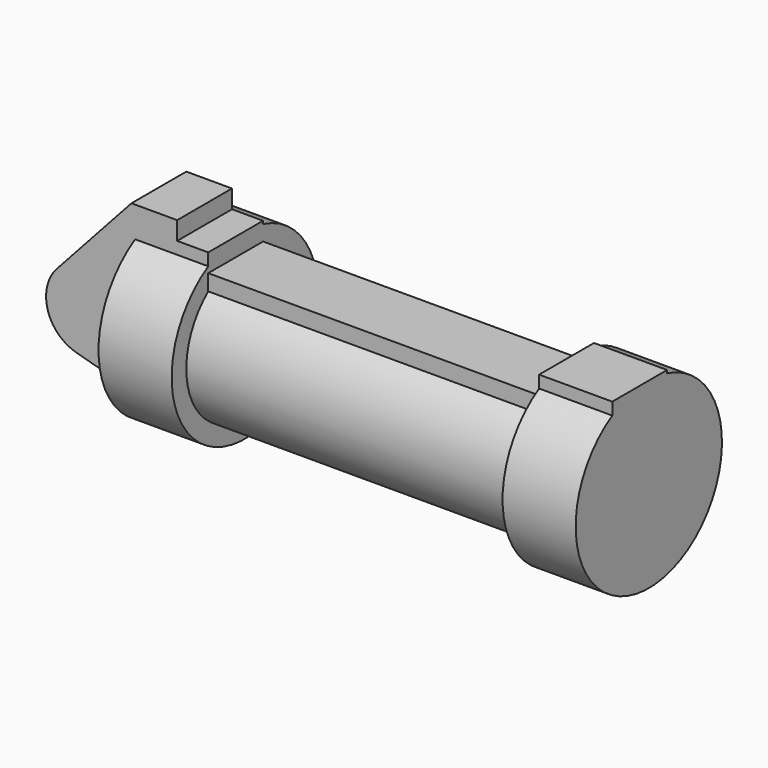
from build123d import *

# Parameters (mm, degrees)
F0_W     = 5.842
F0_H     = 12.7
F0_R     = 3.175
F2_DEPTH = 6.35
F3_DEPTH = 6.35
F4_DEPTH = 3.175
F5_DEPTH = 3.175


# Not quite as in the source:
# - the program builds the solid bodies; features that only make, move or delete a surface that nothing else refers to are left out


with BuildPart() as f1:
    # F0 (on Front) → F1 (revolve)
    with BuildSketch(Plane.XZ):
        Polygon((5.842, 12.7), (5.842, 0), (66.294, 0), (66.294, 12.7), (56.134, 12.7), (56.134, 10.16), (10.16, 10.16), (10.16, 12.7), align=None)
        with Locations((2.921, 6.35)):
            Rectangle(F0_W, F0_H)
    revolve(axis=Axis((33.147, 0, 0), (-1, 0, 0)))

    # F0 (on Front) → F2 (join)
    with BuildSketch(Plane.XZ):
        Polygon((5.842, 12.7), (5.842, 0), (66.294, 0), (66.294, 12.7), (56.134, 12.7), (56.134, 10.16), (10.16, 10.16), (10.16, 12.7), align=None)
        with BuildLine():
            ThreePointArc((-8.1826630726, -5.5069827884), (-3.1957909266, -4.5493385486), (-0.9398, 0))
            ThreePointArc((-0.9398, 0), (-4.5919612295, 5.3297205562), (-10.8806298187, 3.8475430269))
            ThreePointArc((-10.8806298187, 3.8475430269), (-12.1459778134, -1.5837270034), (-8.1826630726, -5.5069827884))
        make_face()
        with Locations((-6.6548, 0)):
            Circle(F0_R, mode=Mode.SUBTRACT)
        with Locations((2.921, 6.35)):
            Rectangle(F0_W, F0_H)
        with BuildLine():
            Line((5.842, 0), (0, 0))
            Line((0, 0), (-0.9398, 0))
            ThreePointArc((-0.9398, 0), (-3.1957909266, -4.5493385486), (-8.1826630726, -5.5069827884))
            Line((-8.1826630726, -5.5069827884), (5.842, -9.398))
            Line((5.842, -9.398), (5.842, 0))
        make_face()
        with Locations((-6.6548, 0)):
            Circle(F0_R)
    extrude(amount=F2_DEPTH)

    # F0 (on Front) → F3 (join)
    with BuildSketch(Plane.XZ):
        with BuildLine():
            Line((-0.9398, 0), (0, 0))
            Line((0, 0), (0, 12.7))
            Line((0, 12.7), (5.842, 12.7))
            Line((5.842, 12.7), (5.842, 15.24))
            Line((5.842, 15.24), (-0.508, 15.24))
            Line((-0.508, 15.24), (-10.8806298187, 3.8475430269))
            ThreePointArc((-10.8806298187, 3.8475430269), (-4.5919612295, 5.3297205562), (-0.9398, 0))
        make_face()
    extrude(amount=F3_DEPTH)

    # F0 (on Front) → F4 (join, symmetric)
    with BuildSketch(Plane.XZ):
        with BuildLine():
            Line((-0.9398, 0), (0, 0))
            Line((0, 0), (0, 12.7))
            Line((0, 12.7), (5.842, 12.7))
            Line((5.842, 12.7), (5.842, 15.24))
            Line((5.842, 15.24), (-0.508, 15.24))
            Line((-0.508, 15.24), (-10.8806298187, 3.8475430269))
            ThreePointArc((-10.8806298187, 3.8475430269), (-4.5919612295, 5.3297205562), (-0.9398, 0))
        make_face()
        with Locations((2.921, 6.35)):
            Rectangle(F0_W, F0_H)
        with BuildLine():
            Line((5.842, 0), (0, 0))
            Line((0, 0), (-0.9398, 0))
            ThreePointArc((-0.9398, 0), (-3.1957909266, -4.5493385486), (-8.1826630726, -5.5069827884))
            Line((-8.1826630726, -5.5069827884), (5.842, -9.398))
            Line((5.842, -9.398), (5.842, 0))
        make_face()
        Polygon((5.842, 12.7), (5.842, 0), (66.294, 0), (66.294, 12.7), (56.134, 12.7), (56.134, 10.16), (10.16, 10.16), (10.16, 12.7), align=None)
        with BuildLine():
            ThreePointArc((-8.1826630726, -5.5069827884), (-3.1957909266, -4.5493385486), (-0.9398, 0))
            ThreePointArc((-0.9398, 0), (-4.5919612295, 5.3297205562), (-10.8806298187, 3.8475430269))
            ThreePointArc((-10.8806298187, 3.8475430269), (-12.1459778134, -1.5837270034), (-8.1826630726, -5.5069827884))
        make_face()
        with Locations((-6.6548, 0)):
            Circle(F0_R, mode=Mode.SUBTRACT)
    extrude(amount=F4_DEPTH, both=True)

    # F0 (on Front) → F5 (join, symmetric)
    with BuildSketch(Plane.XZ):
        Polygon((5.842, 12.7), (5.842, 0), (66.294, 0), (66.294, 12.7), (56.134, 12.7), (56.134, 10.16), (10.16, 10.16), (10.16, 12.7), align=None)
        with BuildLine():
            ThreePointArc((-8.1826630726, -5.5069827884), (-3.1957909266, -4.5493385486), (-0.9398, 0))
            ThreePointArc((-0.9398, 0), (-4.5919612295, 5.3297205562), (-10.8806298187, 3.8475430269))
            ThreePointArc((-10.8806298187, 3.8475430269), (-12.1459778134, -1.5837270034), (-8.1826630726, -5.5069827884))
        make_face()
        with Locations((-6.6548, 0)):
            Circle(F0_R, mode=Mode.SUBTRACT)
        with BuildLine():
            Line((-0.9398, 0), (0, 0))
            Line((0, 0), (0, 12.7))
            Line((0, 12.7), (5.842, 12.7))
            Line((5.842, 12.7), (5.842, 15.24))
            Line((5.842, 15.24), (-0.508, 15.24))
            Line((-0.508, 15.24), (-10.8806298187, 3.8475430269))
            ThreePointArc((-10.8806298187, 3.8475430269), (-4.5919612295, 5.3297205562), (-0.9398, 0))
        make_face()
        with Locations((2.921, 6.35)):
            Rectangle(F0_W, F0_H)
        with BuildLine():
            Line((5.842, 0), (0, 0))
            Line((0, 0), (-0.9398, 0))
            ThreePointArc((-0.9398, 0), (-3.1957909266, -4.5493385486), (-8.1826630726, -5.5069827884))
            Line((-8.1826630726, -5.5069827884), (5.842, -9.398))
            Line((5.842, -9.398), (5.842, 0))
        make_face()
        with Locations((-6.6548, 0)):
            Circle(F0_R)
    extrude(amount=F5_DEPTH, both=True)


solid = f1.part
